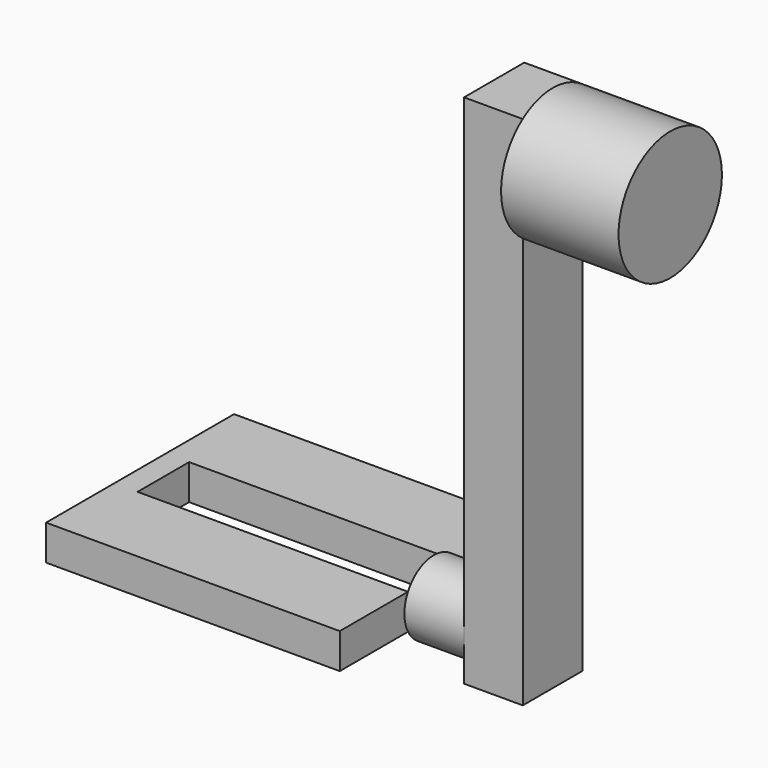
from build123d import *

# Parameters (mm, degrees)
F0_R      = 27.5
F1_DEPTH  = 50
F3_DEPTH  = 25
F4_W      = 25
F4_H      = 31.8995873117
F5_DEPTH  = 175
F6_R      = 15.6245422852
F7_DEPTH  = 25.4
F9_DEPTH  = 125
F10_W     = 115.094
F10_H     = 27.4135967448
F11_DEPTH = 25.4


with BuildPart() as f1:
    # F0 (on Right) → F1 (new body)
    with BuildSketch(Plane.YZ):
        with Locations((20.3808583319, 26.1318925768)):
            Circle(F0_R)
    extrude(amount=F1_DEPTH)

    # F2 (on face) → F3 (join)
    with BuildSketch(Plane(origin=(0, 0, 0), x_dir=(0, -1, 0), z_dir=(-1, 0, 0))):
        with BuildLine():
            ThreePointArc((-36.3306519878, 3.7297926231), (-36.3918107646, 3.7734623502), (-36.4528499765, 3.8172990431))
            Line((-36.4528499765, 3.8172990431), (-36.4528499765, 3.7297926231))
            Line((-36.4528499765, 3.7297926231), (-36.3306519878, 3.7297926231))
        make_face()
        with BuildLine():
            Line((-4.4310646761, 48.4464861105), (-36.4528499765, 48.4464861105))
            Line((-36.4528499765, 48.4464861105), (-36.4528499765, 3.8172990431))
            ThreePointArc((-36.4528499765, 3.8172990431), (-36.3918107646, 3.7734623502), (-36.3306519878, 3.7297926231))
            Line((-36.3306519878, 3.7297926231), (-4.4310646761, 3.7297926231))
            Line((-4.4310646761, 3.7297926231), (-4.4310646761, 48.4464861105))
        make_face()
    extrude(amount=F3_DEPTH)

    # F4 (on face) → F5 (join)
    with BuildSketch(Plane(origin=(0, 0, 3.7297926231), x_dir=(1, 0, 0), z_dir=(0, 0, -1))):
        with Locations((-12.5, -20.3808583319)):
            Rectangle(F4_W, F4_H)
    extrude(amount=F5_DEPTH)


with BuildPart() as f7:
    # F6 (on face) → F7 (new body)
    with BuildSketch(Plane(origin=(-25, 0, 0), x_dir=(0, -1, 0), z_dir=(-1, 0, 0))):
        with Locations((-20.0556069613, -153.3472687006)):
            Circle(F6_R)
    extrude(amount=F7_DEPTH)

    # F8 (on face) → F9 (join)
    with BuildSketch(Plane(origin=(-50.4, 0, 0), x_dir=(0, -1, 0), z_dir=(-1, 0, 0))):
        with BuildLine():
            Line((29.9443930387, -160.8472687006), (29.9443930387, -145.8472687006))
            Line((29.9443930387, -145.8472687006), (-6.3488085888, -145.8472687006))
            ThreePointArc((-6.3488085888, -145.8472687006), (-4.9180911085, -149.4766181831), (-4.4310646761, -153.3472687006))
            ThreePointArc((-4.4310646761, -153.3472687006), (-4.9180911085, -157.2179192181), (-6.3488085888, -160.8472687006))
            Line((-6.3488085888, -160.8472687006), (29.9443930387, -160.8472687006))
        make_face()
        with BuildLine():
            ThreePointArc((-4.4310646761, -153.3472687006), (-4.9180911085, -149.4766181831), (-6.3488085888, -145.8472687006))
            Line((-6.3488085888, -145.8472687006), (-33.7624053337, -145.8472687006))
            ThreePointArc((-33.7624053337, -145.8472687006), (-35.6801492464, -153.3472687006), (-33.7624053337, -160.8472687006))
            Line((-33.7624053337, -160.8472687006), (-6.3488085888, -160.8472687006))
            ThreePointArc((-6.3488085888, -160.8472687006), (-4.9180911085, -157.2179192181), (-4.4310646761, -153.3472687006))
        make_face()
        with BuildLine():
            ThreePointArc((-33.7624053337, -160.8472687006), (-35.6801492464, -153.3472687006), (-33.7624053337, -145.8472687006))
            Line((-33.7624053337, -145.8472687006), (-70.0556069613, -145.8472687006))
            Line((-70.0556069613, -145.8472687006), (-70.0556069613, -160.8472687006))
            Line((-70.0556069613, -160.8472687006), (-33.7624053337, -160.8472687006))
        make_face()
    extrude(amount=F9_DEPTH)

    # F10 (on face) → F11 (cut)
    with BuildSketch(Plane.XY.offset(-145.8472687006)):
        with Locations((-107.947, 20.0556069613)):
            Rectangle(F10_W, F10_H)
    extrude(amount=-F11_DEPTH, mode=Mode.SUBTRACT)


solid = Compound([f1.part, f7.part])
